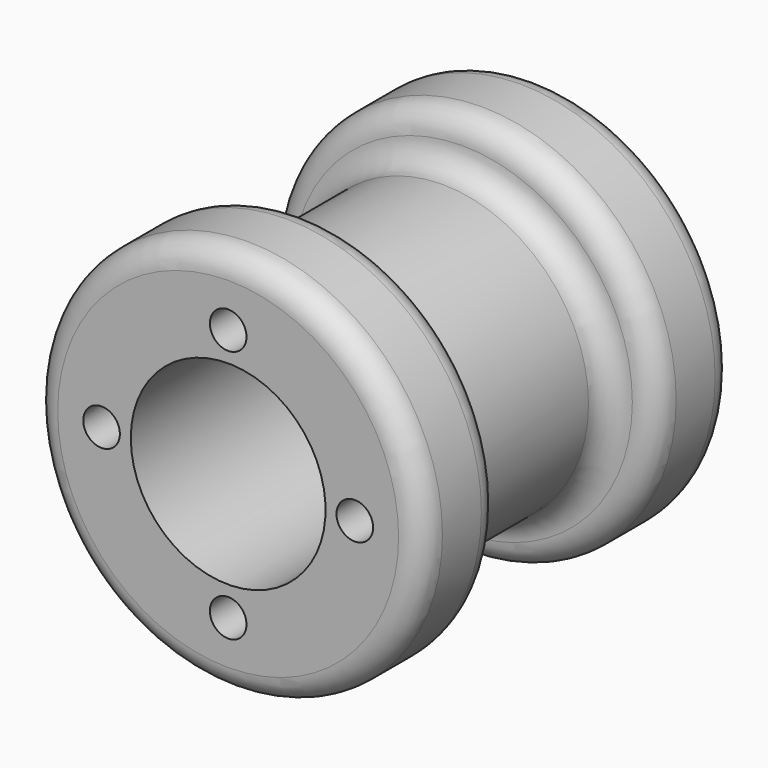
from build123d import *

# Parameters (mm, degrees)
F0_R     = 12.7
F1_DEPTH = 6.35
F2_R     = 9.525
F3_DEPTH = 12.7
F4_R     = 12.7
F4_R_2   = 9.525
F5_DEPTH = 6.35
F7_D     = 12.7
F8_D     = 2.3876
F8_DEPTH = 3.175
F8_TIP   = 0.717307407
F9_R     = 1.58749


# Not quite as in the source:
# - a fillet or chamfer is up to 0.001 mm smaller than in the source, because OpenCascade refuses the exact size


with BuildPart() as f1:
    # F0 (on Front) → F1 (new body)
    with BuildSketch(Plane.XZ):
        Circle(F0_R)
    extrude(amount=F1_DEPTH)

    # F2 (on face) → F3 (join)
    with BuildSketch(Plane.XZ.offset(6.35)):
        Circle(F2_R)
    extrude(amount=F3_DEPTH)

    # F4 (on face) → F5 (join)
    with BuildSketch(Plane.XZ.offset(19.05)):
        Circle(F4_R)
        Circle(F4_R_2, mode=Mode.SUBTRACT)
        Circle(F4_R_2)
    extrude(amount=F5_DEPTH)

    # F7 (through all)
    with Locations(Plane.XZ.offset(25.4)):
        with Locations((0, 0)):
            Hole(F7_D / 2)

    # F8
    with Locations(Plane.XZ.offset(25.4)):
        with Locations((0, 8.255), (-8.255, 0), (0, -8.255), (8.255, 0)):
            Hole(F8_D / 2, depth=F8_DEPTH)
            with Locations((0, 0, -(F8_DEPTH + F8_TIP / 2))):  # 118° drill point
                Cone(0, F8_D / 2, F8_TIP, mode=Mode.SUBTRACT)

    # F9 (radius 1.5875 in the source; OpenCascade refuses exactly that, so slightly less here)
    f9_edges = [f1.edges().sort_by_distance(p)[0] for p in [
        (-12.7, -25.4, 0),
        (-12.7, -19.05, 0),
        (-12.7, -6.35, 0),
        (-12.7, 0, 0),
        (-9.525, -6.35, 0),
        (-9.525, -19.05, 0),
    ]]
    fillet(f9_edges, radius=F9_R)


solid = f1.part
